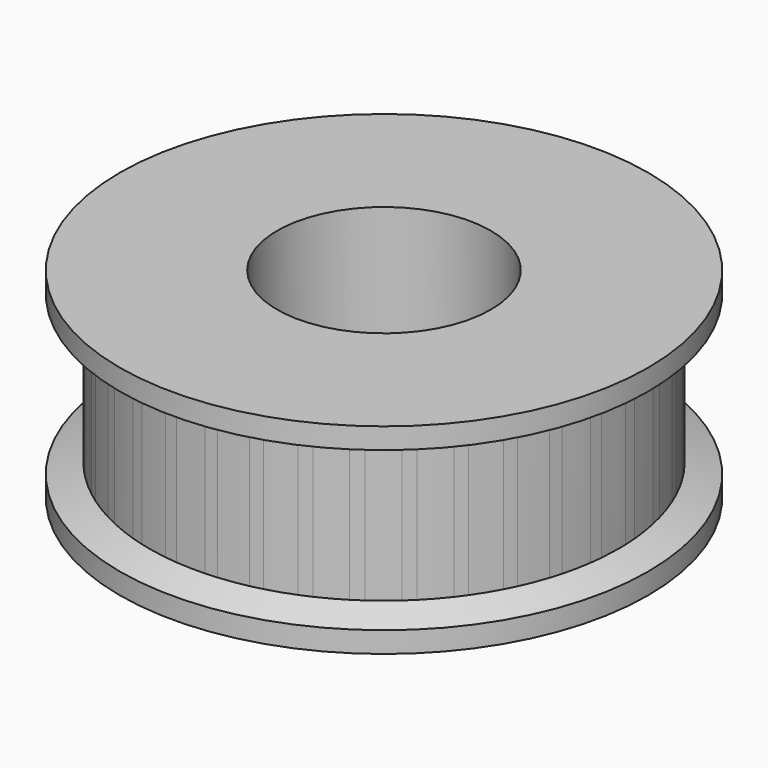
from build123d import *

# Parameters (mm, degrees)
F3_DEPTH = 4.5
F4_COUNT = 36
F7_R     = 5.1
F8_DEPTH = 50


# Not quite as in the source:
# - a feature names something its author has since deleted; it is built from what else it names


with BuildPart() as f3:
    # F2 (on Top) → F3 (new body, symmetric)
    with BuildSketch(Plane.XY):
        with BuildLine():
            Line((0.9112268782, 10.4153708779), (0.9765936853, 11.1625169015))
            ThreePointArc((0.9765936853, 11.1625169015), (0.4887620358, 11.1944910771), (0, 11.2051559026))
            ThreePointArc((0, 11.2051559026), (-0.2034888134, 11.2033080429), (-0.4069105114, 11.1977650733))
            ThreePointArc((-0.4069105114, 11.1977650733), (-0.6919765704, 11.1837689187), (-0.9765936853, 11.1625169015))
            Line((-0.9765936853, 11.1625169015), (-0.9112268782, 10.4153708779))
            Line((-0.9112268782, 10.4153708779), (0, 0))
            Line((0, 0), (0.9112268782, 10.4153708779))
        make_face()
    extrude(amount=F3_DEPTH, both=True)

    # F4: F3 ×36 about axis
    f4_axis = Axis((0, 0, 0), (0, 0, -1))


with BuildPart() as f3_1:
    add(f3.part)
    for i in range(1, F4_COUNT):
        add(f3.part.rotate(f4_axis, i * 360 / F4_COUNT))

    # F5 (on Front) → F6 (revolve)
    with BuildSketch(Plane.XZ):
        Polygon((12.6050714929, 4.5), (0, 4.5), (0, 2.717494719), (10.4551559026, 2.717494719), (12.6050714929, 3.5), align=None)
        Polygon((10.4551559026, -3.282505281), (0, -3.282505281), (0, -5.0650105621), (12.6050714929, -5.0650105621), (12.6050714929, -4.0650105621), align=None)
    revolve(axis=Axis((0, 0, 3.6087473595), (0, 0, 1)))

    # F7 (on Top) → F8 (cut, symmetric)
    with BuildSketch(Plane.XY):
        Circle(F7_R)
    extrude(amount=F8_DEPTH, both=True, mode=Mode.SUBTRACT)


solid = f3_1.part
